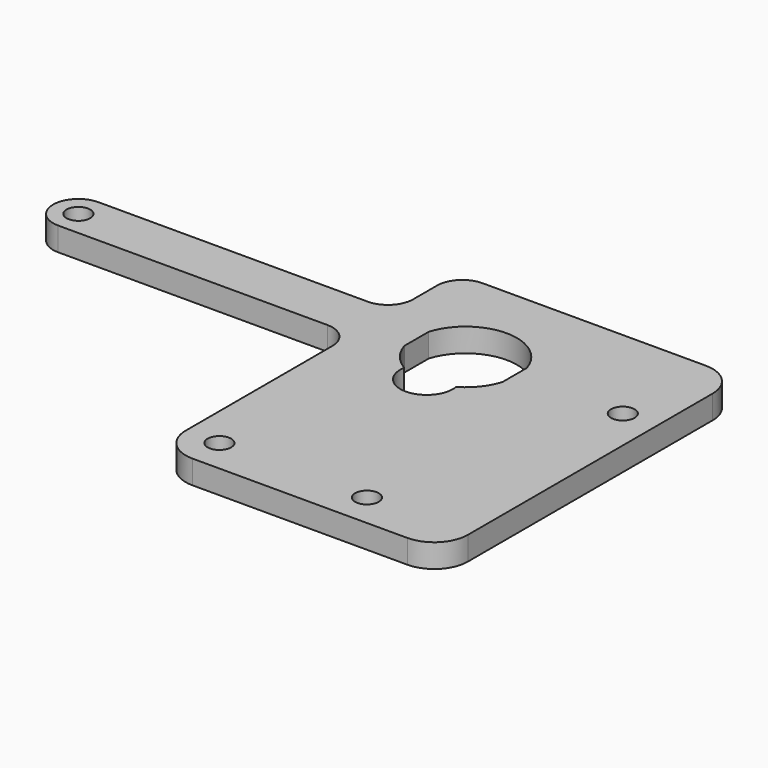
from build123d import *

# Parameters (mm, degrees)
F0_W     = 11.65
F0_H     = 23.75
F1_DEPTH = 20.4
F3_DEPTH = 6
F5_START = -0.8
F4_W     = 11.65
F4_H     = 4.2
F5_DEPTH = 2
F6_R     = 0.5
F7_R     = 1
F8_R     = 1.4
F9_DEPTH = 2.8
F10_R    = 4


# Not quite as in the source:
# - a feature names something its author has since deleted; it is built from what else it names


with BuildPart() as f1:
    # F0 (on Top) → F1 (new body)
    with BuildSketch(Plane.XY):
        Rectangle(F0_W, F0_H)
    extrude(amount=F1_DEPTH)

    # F2 (on face) → F3 (join)
    with BuildSketch(Plane.XY.offset(20.4)):
        with BuildLine():
            Line((5.825, 3.9640955299), (5.825, 7.5859044701))
            ThreePointArc((5.825, 7.5859044701), (0, 11.875), (-5.825, 7.5859044701))
            Line((-5.825, 7.5859044701), (-5.825, 3.9640955299))
            ThreePointArc((-5.825, 3.9640955299), (-4.7781429098, 1.9829886164), (-3.0865775367, 0.5135326087))
            ThreePointArc((-3.0865775367, 0.5135326087), (0, -3.1), (3.0865775367, 0.5135326087))
            ThreePointArc((3.0865775367, 0.5135326087), (4.7781429098, 1.9829886164), (5.825, 3.9640955299))
        make_face()
    extrude(amount=F3_DEPTH)

    # F4 (on face) → F5 (join)
    with BuildSketch(Plane.XY.offset(20.4).offset(F5_START)):
        with Locations((0, -13.975)):
            Rectangle(F4_W, F4_H)
        with Locations((0, 13.975)):
            Rectangle(F4_W, F4_H)
    extrude(amount=-F5_DEPTH)

    # F6
    f6_edges = [f1.edges().sort_by_distance(p)[0] for p in [
        (5.825, 11.875, 8.8),
        (5.825, -11.875, 8.8),
        (-5.825, -11.875, 8.8),
        (-5.825, 11.875, 8.8),
    ]]
    fillet(f6_edges, radius=F6_R)

    # F7
    f7_edges = [f1.edges().sort_by_distance(p)[0] for p in [
        (-5.825, 16.075, 18.6),
        (5.825, 16.075, 18.6),
        (5.825, -16.075, 18.6),
        (-5.825, -16.075, 18.6),
    ]]
    fillet(f7_edges, radius=F7_R)


with BuildPart() as f9:
    # F8 (on face) → F9 (new body)
    with BuildSketch(Plane.XY.offset(26.4)):
        with BuildLine():
            Line((22.5, -26), (22.5, 18.3236394078))
            Line((22.5, 18.3236394078), (1.6129450202, 18.3236394078))
            Line((1.6129450202, 18.3236394078), (-8.0251465812, 18.3236394078))
            ThreePointArc((-8.0251465812, 18.3236394078), (-10.1464669248, 17.4449597513), (-11.0251465812, 15.3236394078))
            Line((-11.0251465812, 15.3236394078), (-11.0251465812, 11.775))
            ThreePointArc((-11.0251465812, 11.775), (-11.9038262377, 9.6536796564), (-14.0251465812, 8.775))
            Line((-14.0251465812, 8.775), (-46, 8.775))
            ThreePointArc((-46, 8.775), (-49, 5.775), (-46, 2.775))
            Line((-46, 2.775), (-14.0251465812, 2.775))
            ThreePointArc((-14.0251465812, 2.775), (-11.9038262377, 1.8963203436), (-11.0251465812, -0.225))
            Line((-11.0251465812, -0.225), (-11.0251465812, -15.0673655123))
            Line((-11.0251465812, -15.0673655123), (-11.0251465812, -26))
            Line((-11.0251465812, -26), (22.5, -26))
        make_face()
        with Locations((-7.0251465812, -22)):
            Circle(F8_R, mode=Mode.SUBTRACT)
        with Locations((10.5, -22)):
            Circle(F8_R, mode=Mode.SUBTRACT)
        with Locations((-46, 5.775)):
            Circle(F8_R, mode=Mode.SUBTRACT)
        with BuildLine():
            ThreePointArc((5.825, 3.9640955299), (4.7781429098, 1.9829886164), (3.0865775367, 0.5135326087))
            ThreePointArc((3.0865775367, 0.5135326087), (0, -3.1290056936), (-3.0865775367, 0.5135326087))
            ThreePointArc((-3.0865775367, 0.5135326087), (-4.7781429098, 1.9829886164), (-5.825, 3.9640955299))
            Line((-5.825, 3.9640955299), (-5.825, 7.5859044701))
            ThreePointArc((-5.825, 7.5859044701), (0, 11.875), (5.825, 7.5859044701))
            Line((5.825, 7.5859044701), (5.825, 3.9640955299))
        make_face(mode=Mode.SUBTRACT)
        with Locations((18.5, 6)):
            Circle(F8_R, mode=Mode.SUBTRACT)
    extrude(amount=-F9_DEPTH)

    # F10
    f10_edges = [f9.edges().sort_by_distance(p)[0] for p in [
        (-11.025147, -26, 25),
        (22.5, -26, 25),
        (22.5, 18.323639, 25),
    ]]
    fillet(f10_edges, radius=F10_R)


with BuildPart() as f11_1:
    # F11: copy of F9
    add(f9.part)


solid = f9.part
